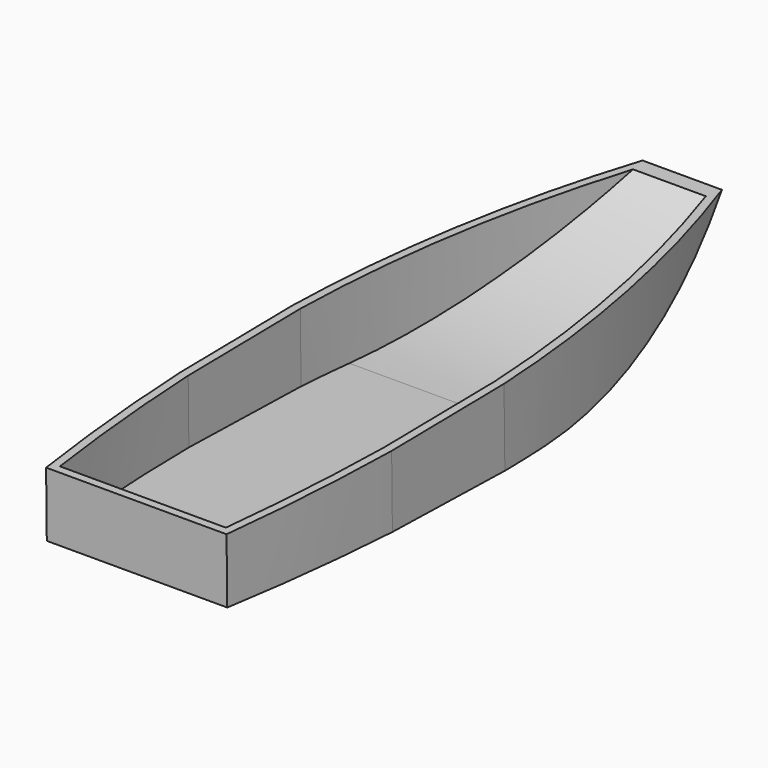
from build123d import *

# Parameters (mm, degrees)
F1_DEPTH = 457.2
F3_DEPTH = 254
F4_T     = 17.78
F5_W     = 50.8
F5_H     = 826.8460257717
F6_DEPTH = 0.508


# Not quite as in the source:
# - a shell that OpenCascade refuses in one call is made with other operations: the cavity is built on its own and cut out


with BuildPart() as f1:
    # F0 (on Right) → F1 (new body)
    with BuildSketch(Plane.YZ):
        with BuildLine():
            Line((288.924485445, -270.4285681248), (-641.1148309708, -283.2744121552))
            Line((-641.1148309708, -283.2744121552), (-641.1148309708, -423.2941567898))
            Line((-641.1148309708, -423.2941567898), (187.4422878027, -442.5629377365))
            ThreePointArc((187.4422878027, -442.5629377365), (523.0417315747, -400.6371692989), (831.9446638759, -262.9282910995))
            Line((831.9446638759, -262.9282910995), (288.924485445, -270.4285681248))
        make_face()
    extrude(amount=F1_DEPTH)

    # F2 (on face) → F3 (cut)
    with BuildSketch(Plane(origin=(0, 3.7895971393, -274.3668944279), x_dir=(1, 0, 0), z_dir=(0, -0.0138108343, 0.9999046259))):
        with BuildLine():
            Line((423.3823697388, -644.965941169), (615.9012913704, -644.965941169))
            Line((615.9012913704, -644.965941169), (483.5176634908, 828.234058831))
            Line((483.5176634908, 828.234058831), (457.2, 61.5478307009))
            ThreePointArc((457.2, 61.5478307009), (455.0788529219, -292.4168742611), (423.3823697388, -644.965941169))
        make_face()
        with BuildLine():
            ThreePointArc((0, 61.5478307009), (43.5944295305, 450.079610673), (142.875, 828.234058831))
            Line((142.875, 828.234058831), (0, 828.234058831))
            Line((0, 828.234058831), (-26.3176634908, 828.234058831))
            Line((-26.3176634908, 828.234058831), (0, 61.5478307009))
        make_face()
        with BuildLine():
            ThreePointArc((33.8176302612, -644.965941169), (2.1211470781, -292.4168742611), (0, 61.5478307009))
            Line((0, 61.5478307009), (-26.3176634908, 828.234058831))
            Line((-26.3176634908, 828.234058831), (-361.6100847721, -644.965941169))
            Line((-361.6100847721, -644.965941169), (33.8176302612, -644.965941169))
        make_face()
        with BuildLine():
            Line((457.2, 61.5478307009), (483.5176634908, 828.234058831))
            Line((483.5176634908, 828.234058831), (457.2, 828.234058831))
            Line((457.2, 828.234058831), (314.325, 828.234058831))
            ThreePointArc((314.325, 828.234058831), (413.6055704695, 450.079610673), (457.2, 61.5478307009))
        make_face()
        Polygon((0, -644.965941169), (-361.6100847721, -644.965941169), (237.2898459435, -852.3167967796), (615.9012913704, -644.965941169), (457.2, -644.965941169), (423.3823697388, -644.965941169), (33.8176302612, -644.965941169), align=None)
    extrude(amount=-F3_DEPTH, mode=Mode.SUBTRACT)

    # F4: shell of thickness 17.78, made by hand


with BuildPart() as f4_core1:
    # F4_t2: copy of F1
    add(f1.part)

    # the walls: a layer under each face that stays
    f4_faces = [f4_core1.faces().sort_by_distance(p)[0] for p in [
        (228.6, 523.0417315747, -400.6371692989),
        (43.5944295305, 455.0197886911, -354.5608330612),
        (413.6055704695, 455.0197886911, -354.5608330612),
        (228.6, -225.8689739056, -432.9510425705),
        (0, -85.1524982143, -356.6467120233),
        (12.0864906617, -438.857755801, -358.0029304556),
        (228.6, -640.1475332924, -353.3067797799),
        (445.1135093383, -438.857755801, -358.0029304556),
        (457.2, -85.1524982143, -356.6467120233),
    ]]
    thicken(f4_faces, amount=-F4_T, mode=Mode.SUBTRACT)


with BuildPart() as f1_1:
    add(f1.part)

    # what is left inside the walls is the cavity
    f4_cavity = [f4_core1.part.solids().sort_by_distance(p)[0] for p in [
        (298.873333, 87.021104, -273.395105),
    ]]
    add(f4_cavity, mode=Mode.SUBTRACT)

    # F5 (on face) → F6 (cut)
    with BuildSketch(Plane(origin=(0, -10.1852834725, -437.9669451445), x_dir=(1, 0, 0), z_dir=(0, -0.0232495407, -0.9997296929))):
        with Locations((103.6994478941, 215.7420070303)):
            Rectangle(F5_W, F5_H)
        with Locations((353.5005521059, 215.7420070303)):
            Rectangle(F5_W, F5_H)
    extrude(amount=-F6_DEPTH, mode=Mode.SUBTRACT)


solid = f1_1.part
